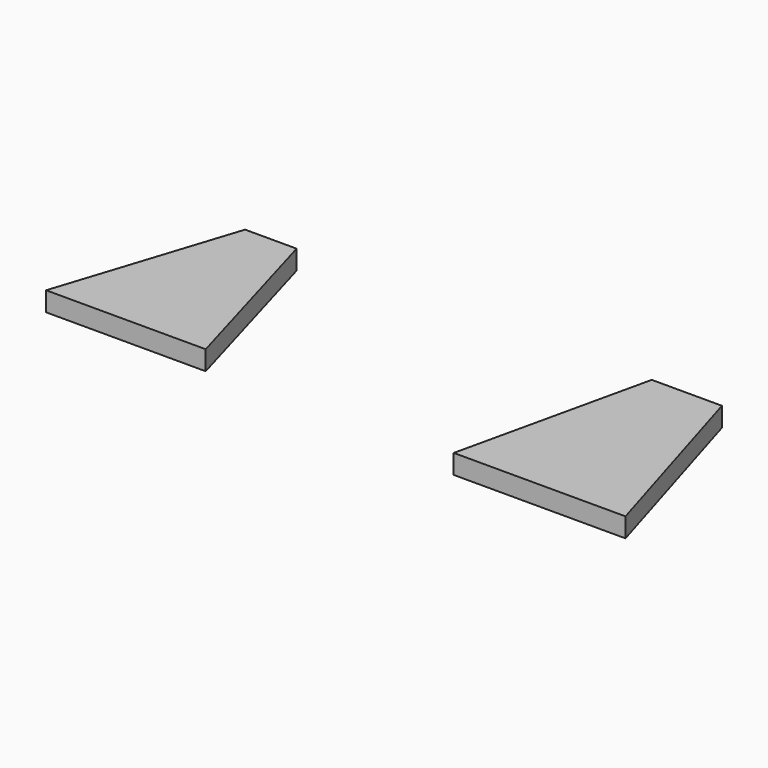
from build123d import *

# Parameters (mm, degrees)
F1_W      = 100
F1_H      = 150
F2_DEPTH  = 3
F4_DEPTH  = 3
F6_DEPTH  = 3
F7_DEPTH  = 184.7764700651
F3_W      = 100
F3_H      = 150
F10_DEPTH = 25
F11_DEPTH = 170.0117439032


# Not quite as in the source:
# - a feature names something its author has since deleted; it is built from what else it names


with BuildPart() as f2:
    # F1 (on face) → F2 (new body)
    with BuildSketch(Plane.XY):
        with Locations((50, 75)):
            Rectangle(F1_W, F1_H)
    extrude(amount=F2_DEPTH)

    # F3 (on face) → F4 (join)
    with BuildSketch(Plane.XY.offset(3)):
        Polygon((38.5150648654, 247.4973201752), (0, 150), (100, 150), align=None)
    extrude(amount=-F4_DEPTH)

    # F5 (on face) → F6 (join)
    with BuildSketch(Plane.XY.offset(3)):
        Polygon((16.8190859258, 0), (8.8544115424, 0), (0, -27.3990668356), (24.6833004057, -27.3990668356), align=None)
        Polygon((82.5879052281, 0), (71.7410296202, 0), (65.0041550398, -29.8579074442), (91.5617346764, -29.8579074442), align=None)
    extrude(amount=-F6_DEPTH)

    # F5 (on face) → F7 (cut)
    with BuildSketch(Plane.XY.offset(3)):
        Polygon((0, 0), (8.8544115424, 0), (16.8190859258, 0), (71.7410296202, 0), (82.5879052281, 0), (100, 0), (100, 150), (38.5150648654, 247.4973201752), (0, 150), align=None)
    extrude(amount=-F7_DEPTH, mode=Mode.SUBTRACT)

    # F3 (on face) → F10 (cut)
    with BuildSketch(Plane.XY.offset(3)):
        with Locations((50, 75)):
            Rectangle(F3_W, F3_H)
    extrude(amount=-F10_DEPTH, mode=Mode.SUBTRACT)

    # F9 (on face) → F11 (cut)
    with BuildSketch(Plane.XY.offset(3)):
        with BuildLine():
            ThreePointArc((71.7517411709, 31.0983583331), (74.2517411709, 28.5983583331), (76.7517411709, 31.0983583331))
            Line((76.7517411709, 31.0983583331), (76.7517411709, 76.4879286289))
            ThreePointArc((76.7517411709, 76.4879286289), (74.2517411709, 78.9879286289), (71.7517411709, 76.4879286289))
            Line((71.7517411709, 76.4879286289), (71.7517411709, 31.0983583331))
        make_face()
    extrude(amount=-F11_DEPTH, mode=Mode.SUBTRACT)


solid = f2.part
